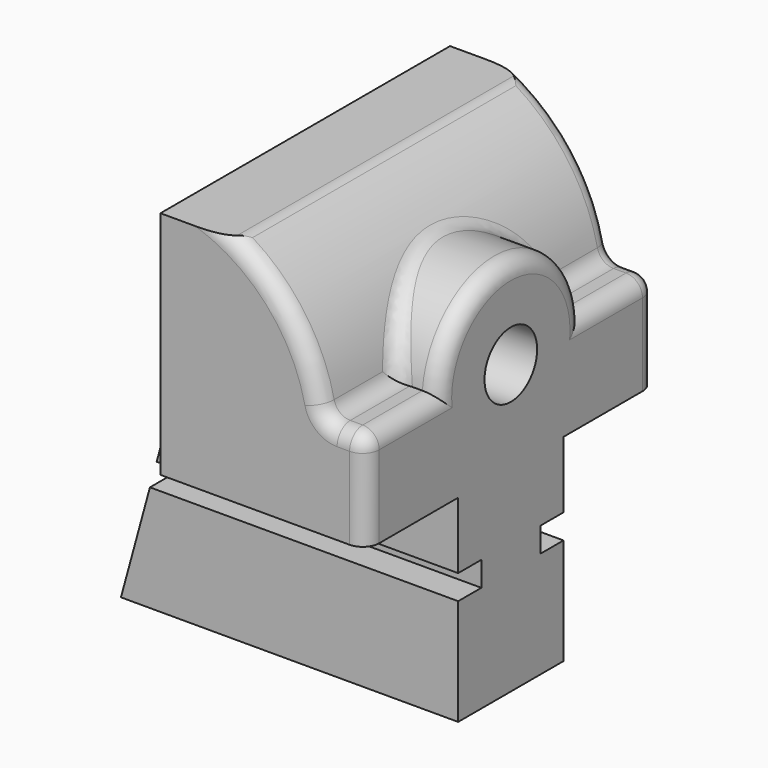
from build123d import *

# Parameters (mm, degrees)
F1_DEPTH = 65.0748
F3_DEPTH = 69.851
F4_R     = 17.4498
F5_DEPTH = 25.4
F6_R     = 6.35
F7_DEPTH = 30.1498
F8_R     = 3.175
F9_DEPTH = 15.875
F10_F1_R = 3.175
F10_F2_R = 3.175


with BuildPart() as f1:
    # F0 (on Right) → F1 (new body)
    with BuildSketch(Plane.YZ):
        Polygon((32.8030504316, 53.1119473694), (-37.0469495684, 53.1119473694), (-37.0469495684, 8.6619473694), (-14.8219495684, 8.6619473694), (-14.8219495684, -4.1650526306), (-9.2339495684, -4.1650526306), (-9.2339495684, -8.9275526306), (-14.8219495684, -8.9275526306), (-14.8219495684, -29.4380526306), (10.5780504316, -29.4380526306), (10.5780504316, -8.9275526306), (4.9900504316, -8.9275526306), (4.9900504316, -4.1650526306), (10.5780504316, -4.1650526306), (10.5780504316, 8.6619473694), (32.8030504316, 8.6619473694), align=None)
    extrude(amount=F1_DEPTH)

    # F2 (on face) → F3 (cut, through all)
    with BuildSketch(Plane.XZ.offset(37.0469495684)):
        with BuildLine():
            ThreePointArc((22.225, 5.4869473694), (24.4700640303, 6.4168833391), (25.4, 8.6619473694))
            Line((25.4, 8.6619473694), (0, 8.6619473694))
            Line((0, 8.6619473694), (0, -29.4380526306))
            Line((0, -29.4380526306), (9.525, 5.4869473694))
            Line((9.525, 5.4869473694), (22.225, 5.4869473694))
        make_face()
        Polygon((25.4, 27.7119473694), (25.4, 53.1119473694), (0, 53.1119473694), (0, 8.6619473694), (25.4, 8.6619473694), align=None)
        with BuildLine():
            Line((65.0748, 53.1119473694), (39.8529659904, 53.1119473694))
            ThreePointArc((39.8529659904, 53.1119473694), (51.2636522621, 42.3660722249), (56.8255061373, 27.7119473694))
            Line((56.8255061373, 27.7119473694), (65.0748, 27.7119473694))
            Line((65.0748, 27.7119473694), (65.0748, 53.1119473694))
        make_face()
    extrude(amount=-F3_DEPTH, mode=Mode.SUBTRACT)

    # F4 (on face) → F5 (join)
    with BuildSketch(Plane.YZ.offset(65.0748)):
        with Locations((-2.1219495684, 26.1117473694)):
            Circle(F4_R)
    extrude(amount=-F5_DEPTH)

    # F6 (on face) → F7 (cut)
    with BuildSketch(Plane.YZ.offset(65.0748)):
        with Locations((-2.1219495684, 26.1117473694)):
            Circle(F6_R)
    extrude(amount=-F7_DEPTH, mode=Mode.SUBTRACT)

    # F8 (on face) → F9 (cut)
    with BuildSketch(Plane(origin=(25.4, 0, 0), x_dir=(0, -1, 0), z_dir=(-1, 0, 0))):
        with Locations((-16.9280504316, 34.0619473694)):
            Circle(F8_R)
        with Locations((21.1719495684, 34.0619473694)):
            Circle(F8_R)
    extrude(amount=-F9_DEPTH, mode=Mode.SUBTRACT)

    # F10: fillet of radius 3.175 on 12 edges, made by hand

    # F10_f1
    f10_f1_edges = [f1.edges().sort_by_distance(p)[0] for p in [
        (50.428197841, -2.1264417395, 43.5615467912),
        (56.8255061373, -28.2725863076, 27.7119473694),
        (56.8255061373, 24.0286871709, 27.7119473694),
    ]]
    fillet(f10_f1_edges, radius=F10_F1_R)

    # F10_f2
    f10_f2_edges = [f1.edges().sort_by_distance(p)[0] for p in [
        (50.5351306509, -37.0469495684, 43.4143386342),
        (62.2832541328, -37.0469495684, 27.7119473694),
        (65.0748, 32.8030504316, 18.1869473694),
        (50.5351306509, 32.8030504316, 43.4143386342),
        (39.8529659904, -2.1219495684, 53.1119473694),
        (65.0748, -28.2725863076, 27.7119473694),
        (65.0748, -2.1219495684, 43.5615473694),
        (65.0748, 24.0286871709, 27.7119473694),
        (65.0748, -37.0469495684, 18.1869473694),
        (57.4937274099, 32.8030504316, 28.4194187475),
        (57.4937274099, -37.0469495684, 28.4194187475),
    ]]
    fillet(f10_f2_edges, radius=F10_F2_R)


solid = f1.part
